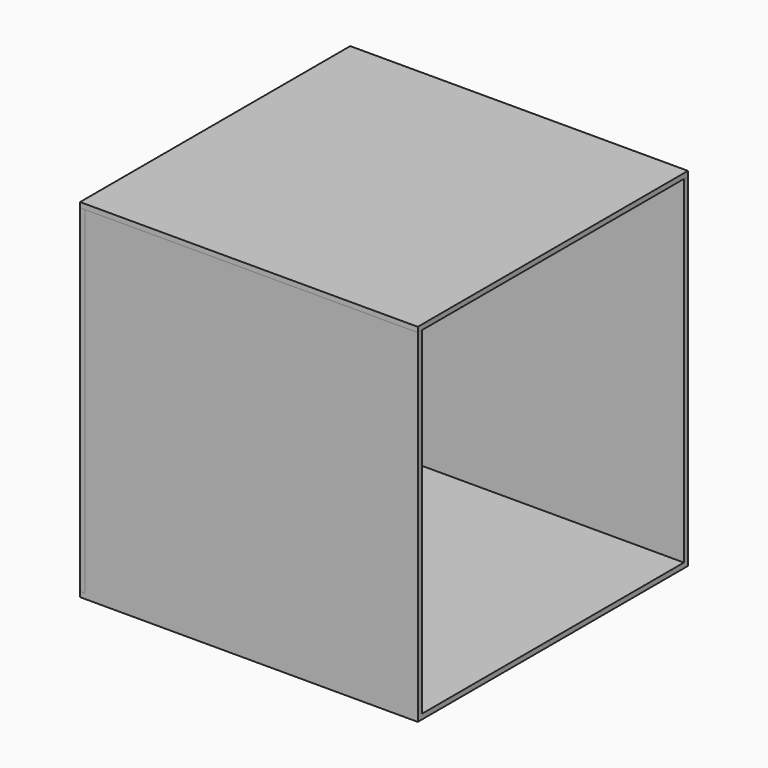
from build123d import *

# Parameters (mm, degrees)
F0_W     = 600
F0_H     = 600
F1_DEPTH = 9
F2_W     = 9
F2_H     = 600
F3_DEPTH = 600
F4_W     = 591
F4_H     = 9
F5_DEPTH = 600
F6_W     = 591
F6_H     = 9
F7_DEPTH = 600
F8_W     = 600.0019320287
F8_H     = 599.9984145164
F9_DEPTH = 9


with BuildPart() as f1:
    # F0 (on Top) → F1 (new body)
    with BuildSketch(Plane.XY):
        with Locations((305.9059588239, 300)):
            Rectangle(F0_W, F0_H)
    extrude(amount=F1_DEPTH)

    # F4 (on face) → F5 (join)
    with BuildSketch(Plane.XY.offset(9)):
        with Locations((310.4059588239, 595.5)):
            Rectangle(F4_W, F4_H)
    extrude(amount=F5_DEPTH)

    # F6 (on face) → F7 (join)
    with BuildSketch(Plane.XY.offset(9)):
        with Locations((310.4059588239, 4.5)):
            Rectangle(F6_W, F6_H)
    extrude(amount=F7_DEPTH)


with BuildPart() as f3:
    # F2 (on face) → F3 (new body)
    with BuildSketch(Plane.XY.offset(9)):
        with Locations((10.4059588239, 300)):
            Rectangle(F2_W, F2_H)
    extrude(amount=F3_DEPTH)


with BuildPart() as f9:
    # F8 (on face) → F9 (new body)
    with BuildSketch(Plane.XY.offset(609)):
        with Locations((305.9049928095, 299.9992072582)):
            Rectangle(F8_W, F8_H)
    extrude(amount=F9_DEPTH)


solid = Compound([f1.part, f3.part, f9.part])
